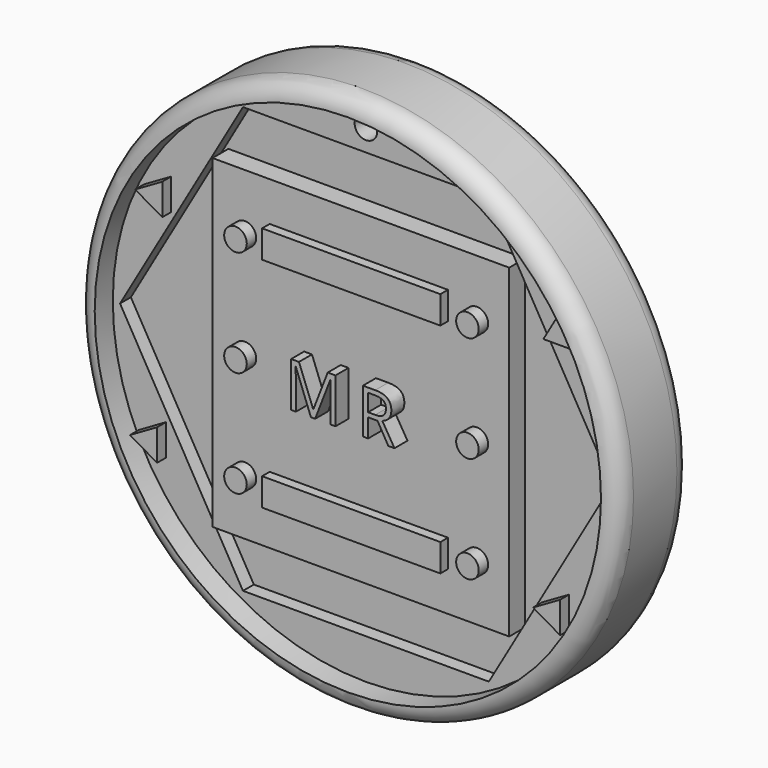
from build123d import *

# Parameters (mm, degrees)
F0_R         = 76.2
F1_DEPTH     = 25.4
F2_R         = 5.08
F3_DEPTH     = 6.35
F7_D         = 6.35
F8_R         = 3.175
F9_DEPTH     = 5.08
F11_DEPTH    = 20.32
F12_W        = 83.3619683981
F12_H        = 91.2318006158
F13_DEPTH    = 20.828
F15_DEPTH    = 22.098
F17_DEPTH    = 22.098
F19_DEPTH    = 22.098
F21_DEPTH    = 22.098
F24_W        = 50.0888
F24_H        = 7.7707562596
F25_DEPTH    = 3.175
F4_TEXT_SIZE = 17.6388888889
F26_DEPTH    = 6.35
F5_TEXT_SIZE = 17.6388888889
F27_DEPTH    = 6.35
F28_DEPTH    = 5.08


# Not quite as in the source:
# - the program builds the solid bodies; features that only make, move or delete a surface that nothing else refers to are left out
# - Text() gives the source's letters only with a copy of the font that has no kerning and outlines rounded to 1/6400 em; it was checked with that copy


with BuildPart() as f1:
    # F0 (on Front) → F1 (new body)
    with BuildSketch(Plane.XZ):
        Circle(F0_R)
    extrude(amount=F1_DEPTH)

    # F2
    f2_edges = [f1.edges().sort_by_distance(p)[0] for p in [
        (-76.2, -25.4, 0),
        (-76.2, 0, 0),
    ]]
    fillet(f2_edges, radius=F2_R)

    # F3 (cut): a face of the model
    f3_faces = [f1.faces().sort_by_distance(p)[0] for p in [
        (0, -25.4, 0),
    ]]
    extrude(f3_faces, amount=-F3_DEPTH, mode=Mode.SUBTRACT)

    # F7 (through all)
    with Locations(Plane(origin=(0, 0, 0), x_dir=(1, 0, 0), z_dir=(0, 1, 0))):
        with Locations((0, -66.04)):
            Hole(F7_D / 2)

    # F10 (on Front) → F11 (join)
    with BuildSketch(Plane.XZ):
        Polygon((69.0796747804, 0), (34.5398373902, 59.824753245), (-34.5398373902, 59.824753245), (-69.0796747804, 0), (-34.5398373902, -59.824753245), (34.5398373902, -59.824753245), align=None)
    extrude(amount=F11_DEPTH)

    # F12 (on Front) → F13 (join)
    with BuildSketch(Plane.XZ):
        Rectangle(F12_W, F12_H)
    extrude(amount=F13_DEPTH)

    # F14 (on Front) → F15 (join)
    with BuildSketch(Plane.XZ):
        Polygon((52.2940521325, 31.9165587425), (61.3813559328, 31.9165587425), (56.8377040327, 39.7863946855), align=None)
    extrude(amount=F15_DEPTH)

    # F16 (on Front) → F17 (join)
    with BuildSketch(Plane.XZ):
        Polygon((57.0042583621, -39.8136726573), (57.0042583621, -31.0148545548), (49.3842583621, -35.4142636061), align=None)
    extrude(amount=F17_DEPTH)

    # F18 (on Front) → F19 (join)
    with BuildSketch(Plane.XZ):
        Polygon((-54.7765601897, 27.2256718025), (-54.7765601897, 36.0244899049), (-62.3965601897, 31.6250808537), align=None)
    extrude(amount=F19_DEPTH)

    # F20 (on Front) → F21 (join)
    with BuildSketch(Plane.XZ):
        Polygon((-56.23393287, -33.9841633096), (-56.23393287, -25.1853452072), (-63.85393287, -29.5847542584), align=None)
    extrude(amount=F21_DEPTH)

    # F24 (on face) → F25 (join)
    with BuildSketch(Plane.XZ.offset(20.32)):
        with Locations((-0.57031425, 30.6513113901)):
            Rectangle(F24_W, F24_H)
        with Locations((-0.57031425, -30.6513113901)):
            Rectangle(F24_W, F24_H)
    extrude(amount=F25_DEPTH)

    # F4 (on face) → F26 (join)
    with BuildSketch(Plane.XZ.offset(19.05)):
        with Locations((-17.6693197053, -6.4538134027)):
            Text('M', F4_TEXT_SIZE, font='Open Sans', text_align=(TextAlign.LEFT, TextAlign.BOTTOM))
    extrude(amount=F26_DEPTH)

    # F5 (on face) → F27 (join)
    with BuildSketch(Plane.XZ.offset(19.05)):
        with Locations((2.502649255, -6.4819689217)):
            Text('R', F5_TEXT_SIZE, font='Open Sans', text_align=(TextAlign.LEFT, TextAlign.BOTTOM))
    extrude(amount=F27_DEPTH)

    # F28 (cut): a face of the model
    f28_faces = [f1.faces().sort_by_distance(p)[0] for p in [
        (50.226941892, -20.32, 28.9985384219),
    ]]
    extrude(f28_faces, amount=-F28_DEPTH, mode=Mode.SUBTRACT)


with BuildPart() as f9:
    # F8 (on face) → F9 (new body)
    with BuildSketch(Plane.XZ.offset(19.05)):
        with Locations((-32.586231617, -29.8125877516)):
            Circle(F8_R)
    extrude(amount=F9_DEPTH)


with BuildPart() as f9b:
    # F8 (on face) → F9, piece 2 (new body)
    with BuildSketch(Plane.XZ.offset(19.05)):
        with Locations((-32.586231617, 0)):
            Circle(F8_R)
    extrude(amount=F9_DEPTH)


with BuildPart() as f9c:
    # F8 (on face) → F9, piece 3 (new body)
    with BuildSketch(Plane.XZ.offset(19.05)):
        with Locations((-32.586231617, 29.8196)):
            Circle(F8_R)
    extrude(amount=F9_DEPTH)


with BuildPart() as f9d:
    # F8 (on face) → F9, piece 4 (new body)
    with BuildSketch(Plane.XZ.offset(19.05)):
        with Locations((32.5882, -29.8196)):
            Circle(F8_R)
    extrude(amount=F9_DEPTH)


with BuildPart() as f9e:
    # F8 (on face) → F9, piece 5 (new body)
    with BuildSketch(Plane.XZ.offset(19.05)):
        with Locations((32.5882, 0)):
            Circle(F8_R)
    extrude(amount=F9_DEPTH)


with BuildPart() as f9f:
    # F8 (on face) → F9, piece 6 (new body)
    with BuildSketch(Plane.XZ.offset(19.05)):
        with Locations((32.5882, 29.8196)):
            Circle(F8_R)
    extrude(amount=F9_DEPTH)


solid = Compound([f1.part, f9.part, f9b.part, f9c.part, f9d.part, f9e.part, f9f.part])
